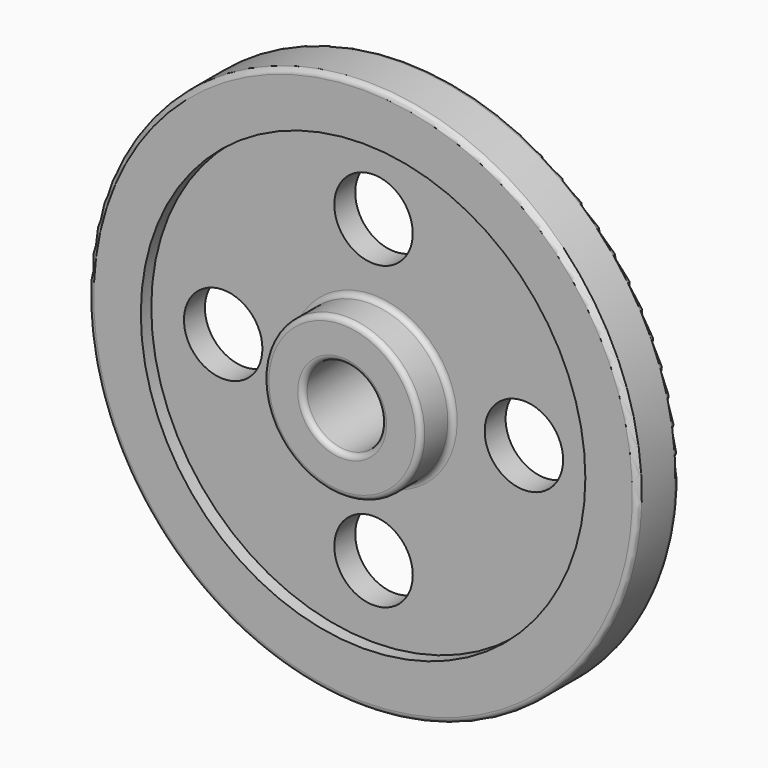
from build123d import *

# Parameters (mm, degrees)
F2_R     = 19.05
F3_DEPTH = 25.4
F4_R     = 2.54
F5_SIZE  = 1.6002


with BuildPart() as f1:
    # F0 (on Right) → F1 (revolve)
    with BuildSketch(Plane.YZ):
        Polygon((-12.7, 19.05), (0, 19.05), (12.7, 19.05), (25.4, 19.05), (25.4, 38.1), (12.7, 38.1), (6.35, 38.1), (6.35, 107.95), (12.7, 107.95), (12.7, 133.35), (0, 133.35), (-12.7, 133.35), (-12.7, 107.95), (-6.35, 107.95), (-6.35, 38.1), (-12.7, 38.1), (-25.4, 38.1), (-25.4, 19.05), align=None)
    revolve(axis=Axis((0, 37.7952009439, 0), (0, 1, 0)))

    # F2 (on face) → F3 (cut)
    with BuildSketch(Plane.XZ.offset(6.35)):
        with Locations((-73.025, 0)):
            Circle(F2_R)
        with Locations((0, -73.025)):
            Circle(F2_R)
        with Locations((73.025, 0)):
            Circle(F2_R)
        with BuildLine():
            ThreePointArc((19.05, 73.025), (-13.4703841816, 86.4953841816), (0, 53.975))
            ThreePointArc((0, 53.975), (13.4703841816, 59.5546158184), (19.05, 73.025))
        make_face()
    extrude(amount=-F3_DEPTH, mode=Mode.SUBTRACT)

    # F4
    f4_edges = [f1.edges().sort_by_distance(p)[0] for p in [
        (0, -6.35, -38.1),
        (0, -15.875, 38.1),
        (0, -25.4, -38.1),
        (0, -25.4, -19.05),
        (0, 25.4, -38.1),
        (0, 15.875, 38.1),
        (0, 6.35, -38.1),
        (0, -12.7, -133.35),
        (0, 12.7, -133.35),
    ]]
    fillet(f4_edges, radius=F4_R)

    # F5
    f5_edges = [f1.edges().sort_by_distance(p)[0] for p in [
        (0, 25.4, -19.05),
    ]]
    chamfer(f5_edges, length=F5_SIZE)


solid = f1.part
